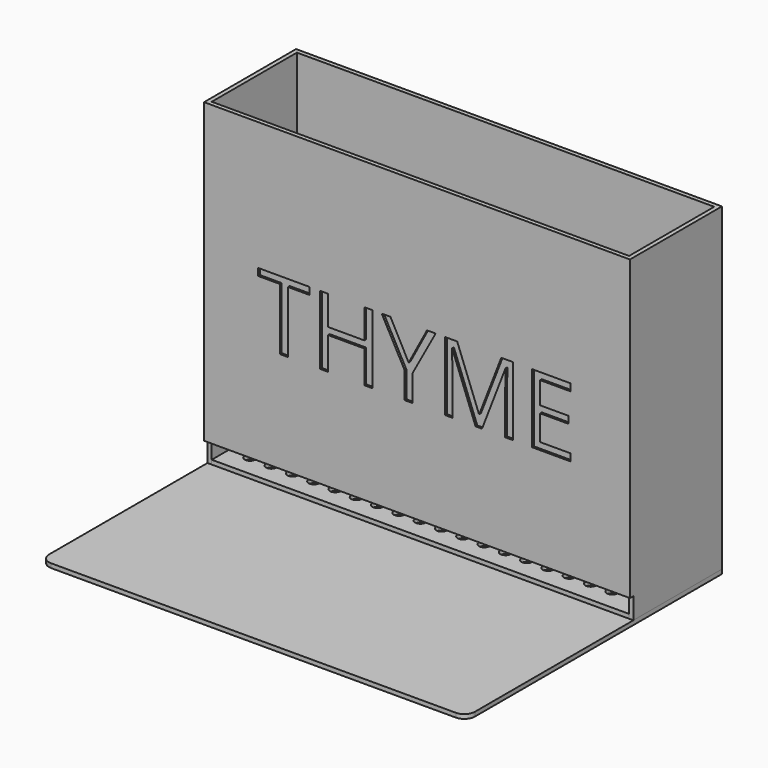
from build123d import *

# Parameters (mm, degrees)
F0_W         = 200
F0_H         = 150
F1_DEPTH     = 2
F2_W         = 2
F2_H         = 50
F3_DEPTH     = 150
F5_W         = 196
F5_H         = 50
F5_R         = 2.5
F6_DEPTH     = 2
F4_TEXT_SIZE = 45.2510016498
F7_DEPTH     = 1
F8_R         = 5
F9_R         = 5
F10_W        = 200
F10_H        = 10
F11_DEPTH    = 2


# Not quite as in the source:
# - Text() gives the source's letters only with a copy of the font that has no kerning and outlines rounded to 1/6400 em; it was checked with that copy


with BuildPart() as f1:
    # F0 (on Top) → F1 (new body)
    with BuildSketch(Plane.XY):
        with Locations((100, -75)):
            Rectangle(F0_W, F0_H)
    extrude(amount=F1_DEPTH)

    # F8
    f8_edges = [f1.edges().sort_by_distance(p)[0] for p in [
        (200, -150, 1),
    ]]
    fillet(f8_edges, radius=F8_R)

    # F9
    f9_edges = [f1.edges().sort_by_distance(p)[0] for p in [
        (0, -150, 1),
    ]]
    fillet(f9_edges, radius=F9_R)


with BuildPart() as f3:
    # F2 (on face) → F3 (new body)
    with BuildSketch(Plane.XY.offset(2)):
        Polygon((200, 0), (0, 0), (0, -2), (2, -2), (198, -2), (200, -2), align=None)
        with Locations((1, -27)):
            Rectangle(F2_W, F2_H)
        with Locations((199, -27)):
            Rectangle(F2_W, F2_H)
        Polygon((2, -52), (0, -52), (0, -54), (200, -54), (200, -52), (198, -52), align=None)
    extrude(amount=F3_DEPTH)

    # F4 (on face) → F7 (cut)
    with BuildSketch(Plane.XZ.offset(54)):
        with Locations((25, 59.4192788122)):
            Text('THYME', F4_TEXT_SIZE, font='Open Sans', text_align=(TextAlign.LEFT, TextAlign.BOTTOM))
    extrude(amount=-F7_DEPTH, mode=Mode.SUBTRACT)

    # F10 (on face) → F11 (cut)
    with BuildSketch(Plane.XZ.offset(54)):
        with Locations((100, 7)):
            Rectangle(F10_W, F10_H)
    extrude(amount=-F11_DEPTH, mode=Mode.SUBTRACT)


with BuildPart() as f6:
    # F5 (on face) → F6 (new body)
    with BuildSketch(Plane.XY.offset(2)):
        with Locations((100, -27)):
            Rectangle(F5_W, F5_H)
        with Locations((12, -42)):
            Circle(F5_R, mode=Mode.SUBTRACT)
        with Locations((22, -42)):
            Circle(F5_R, mode=Mode.SUBTRACT)
        with Locations((32, -42)):
            Circle(F5_R, mode=Mode.SUBTRACT)
        with Locations((42, -42)):
            Circle(F5_R, mode=Mode.SUBTRACT)
        with Locations((52, -42)):
            Circle(F5_R, mode=Mode.SUBTRACT)
        with Locations((62, -42)):
            Circle(F5_R, mode=Mode.SUBTRACT)
        with Locations((72, -42)):
            Circle(F5_R, mode=Mode.SUBTRACT)
        with Locations((82, -42)):
            Circle(F5_R, mode=Mode.SUBTRACT)
        with Locations((92, -42)):
            Circle(F5_R, mode=Mode.SUBTRACT)
        with Locations((12, -32)):
            Circle(F5_R, mode=Mode.SUBTRACT)
        with Locations((22, -32)):
            Circle(F5_R, mode=Mode.SUBTRACT)
        with Locations((32, -32)):
            Circle(F5_R, mode=Mode.SUBTRACT)
        with Locations((42, -32)):
            Circle(F5_R, mode=Mode.SUBTRACT)
        with Locations((52, -32)):
            Circle(F5_R, mode=Mode.SUBTRACT)
        with Locations((62, -32)):
            Circle(F5_R, mode=Mode.SUBTRACT)
        with Locations((72, -32)):
            Circle(F5_R, mode=Mode.SUBTRACT)
        with Locations((82, -32)):
            Circle(F5_R, mode=Mode.SUBTRACT)
        with Locations((92, -32)):
            Circle(F5_R, mode=Mode.SUBTRACT)
        with Locations((102, -42)):
            Circle(F5_R, mode=Mode.SUBTRACT)
        with Locations((112, -42)):
            Circle(F5_R, mode=Mode.SUBTRACT)
        with Locations((122, -42)):
            Circle(F5_R, mode=Mode.SUBTRACT)
        with Locations((132, -42)):
            Circle(F5_R, mode=Mode.SUBTRACT)
        with Locations((142, -42)):
            Circle(F5_R, mode=Mode.SUBTRACT)
        with Locations((152, -42)):
            Circle(F5_R, mode=Mode.SUBTRACT)
        with Locations((162, -42)):
            Circle(F5_R, mode=Mode.SUBTRACT)
        with Locations((172, -42)):
            Circle(F5_R, mode=Mode.SUBTRACT)
        with Locations((182, -42)):
            Circle(F5_R, mode=Mode.SUBTRACT)
        with Locations((102, -32)):
            Circle(F5_R, mode=Mode.SUBTRACT)
        with Locations((112, -32)):
            Circle(F5_R, mode=Mode.SUBTRACT)
        with Locations((122, -32)):
            Circle(F5_R, mode=Mode.SUBTRACT)
        with Locations((132, -32)):
            Circle(F5_R, mode=Mode.SUBTRACT)
        with Locations((142, -32)):
            Circle(F5_R, mode=Mode.SUBTRACT)
        with Locations((152, -32)):
            Circle(F5_R, mode=Mode.SUBTRACT)
        with Locations((162, -32)):
            Circle(F5_R, mode=Mode.SUBTRACT)
        with Locations((172, -32)):
            Circle(F5_R, mode=Mode.SUBTRACT)
        with Locations((182, -32)):
            Circle(F5_R, mode=Mode.SUBTRACT)
        with Locations((12, -22)):
            Circle(F5_R, mode=Mode.SUBTRACT)
        with Locations((22, -22)):
            Circle(F5_R, mode=Mode.SUBTRACT)
        with Locations((32, -22)):
            Circle(F5_R, mode=Mode.SUBTRACT)
        with Locations((42, -22)):
            Circle(F5_R, mode=Mode.SUBTRACT)
        with Locations((52, -22)):
            Circle(F5_R, mode=Mode.SUBTRACT)
        with Locations((62, -22)):
            Circle(F5_R, mode=Mode.SUBTRACT)
        with Locations((72, -22)):
            Circle(F5_R, mode=Mode.SUBTRACT)
        with Locations((82, -22)):
            Circle(F5_R, mode=Mode.SUBTRACT)
        with Locations((92, -22)):
            Circle(F5_R, mode=Mode.SUBTRACT)
        with Locations((12, -12)):
            Circle(F5_R, mode=Mode.SUBTRACT)
        with Locations((22, -12)):
            Circle(F5_R, mode=Mode.SUBTRACT)
        with Locations((32, -12)):
            Circle(F5_R, mode=Mode.SUBTRACT)
        with Locations((42, -12)):
            Circle(F5_R, mode=Mode.SUBTRACT)
        with Locations((52, -12)):
            Circle(F5_R, mode=Mode.SUBTRACT)
        with Locations((62, -12)):
            Circle(F5_R, mode=Mode.SUBTRACT)
        with Locations((72, -12)):
            Circle(F5_R, mode=Mode.SUBTRACT)
        with Locations((82, -12)):
            Circle(F5_R, mode=Mode.SUBTRACT)
        with Locations((92, -12)):
            Circle(F5_R, mode=Mode.SUBTRACT)
        with Locations((102, -22)):
            Circle(F5_R, mode=Mode.SUBTRACT)
        with Locations((112, -22)):
            Circle(F5_R, mode=Mode.SUBTRACT)
        with Locations((122, -22)):
            Circle(F5_R, mode=Mode.SUBTRACT)
        with Locations((132, -22)):
            Circle(F5_R, mode=Mode.SUBTRACT)
        with Locations((142, -22)):
            Circle(F5_R, mode=Mode.SUBTRACT)
        with Locations((152, -22)):
            Circle(F5_R, mode=Mode.SUBTRACT)
        with Locations((162, -22)):
            Circle(F5_R, mode=Mode.SUBTRACT)
        with Locations((172, -22)):
            Circle(F5_R, mode=Mode.SUBTRACT)
        with Locations((182, -22)):
            Circle(F5_R, mode=Mode.SUBTRACT)
        with Locations((102, -12)):
            Circle(F5_R, mode=Mode.SUBTRACT)
        with Locations((112, -12)):
            Circle(F5_R, mode=Mode.SUBTRACT)
        with Locations((122, -12)):
            Circle(F5_R, mode=Mode.SUBTRACT)
        with Locations((132, -12)):
            Circle(F5_R, mode=Mode.SUBTRACT)
        with Locations((142, -12)):
            Circle(F5_R, mode=Mode.SUBTRACT)
        with Locations((152, -12)):
            Circle(F5_R, mode=Mode.SUBTRACT)
        with Locations((162, -12)):
            Circle(F5_R, mode=Mode.SUBTRACT)
        with Locations((172, -12)):
            Circle(F5_R, mode=Mode.SUBTRACT)
        with Locations((182, -12)):
            Circle(F5_R, mode=Mode.SUBTRACT)
    extrude(amount=F6_DEPTH)


solid = Compound([f1.part, f3.part, f6.part])
